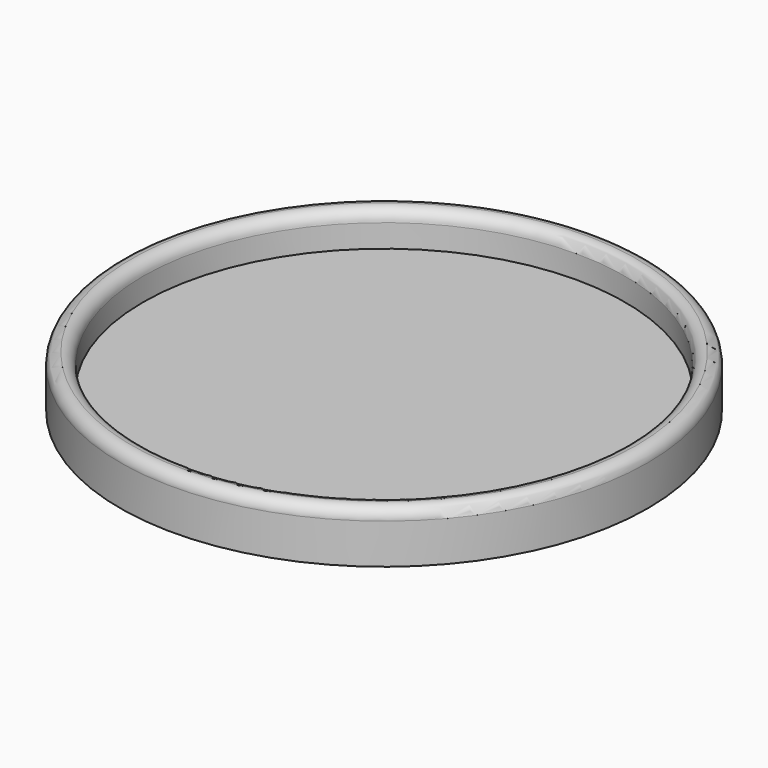
from build123d import *

# Parameters (mm, degrees)
F0_R     = 23
F0_R_2   = 21
F1_DEPTH = 4.5
F2_DEPTH = 3
F3_R     = 0.99999


# Not quite as in the source:
# - a fillet or chamfer is up to 0.001 mm smaller than in the source, because OpenCascade refuses the exact size


with BuildPart() as f1:
    # F0 (on Top) → F1 (new body)
    with BuildSketch(Plane.XY):
        Circle(F0_R)
        Circle(F0_R_2, mode=Mode.SUBTRACT)
        Circle(F0_R_2)
    extrude(amount=-F1_DEPTH)

    # F0 (on Top) → F2 (cut)
    with BuildSketch(Plane.XY):
        Circle(F0_R_2)
    extrude(amount=-F2_DEPTH, mode=Mode.SUBTRACT)

    # F3 (radius 1 in the source; OpenCascade refuses exactly that, so slightly less here)
    f3_edges = [f1.edges().sort_by_distance(p)[0] for p in [
        (-21, 0, 0),
        (-23, 0, 0),
    ]]
    fillet(f3_edges, radius=F3_R)


solid = f1.part
